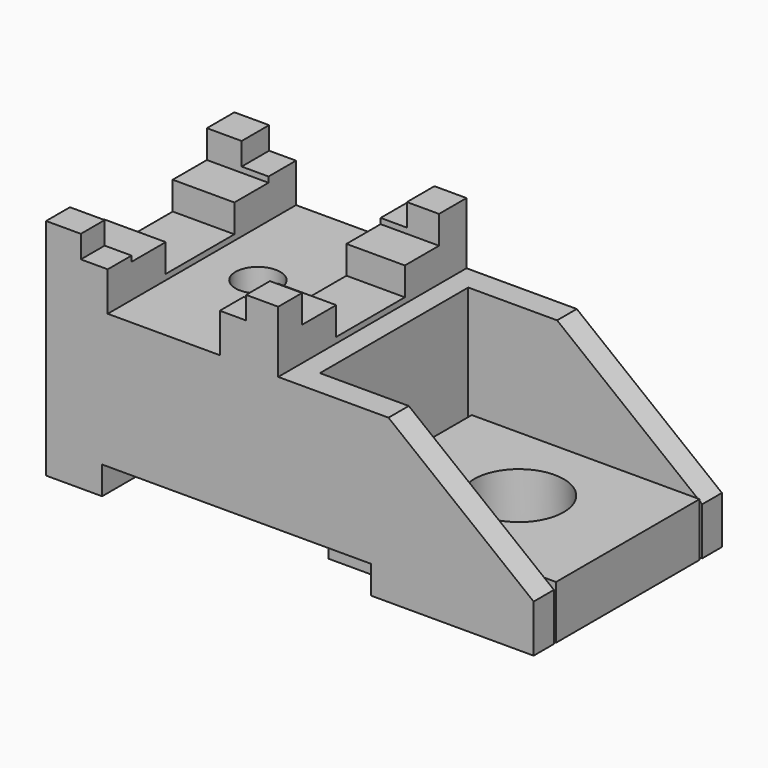
from build123d import *

# Parameters (mm, degrees)
F0_W      = 43.5
F0_H      = 20
F1_DEPTH  = 21
F2_W      = 24
F2_H      = 2.5
F2_W_2    = 2.3986939639
F2_H_2    = 2.0085112005
F2_W_3    = 2.3467258811
F3_DEPTH  = 21.001
F5_DEPTH  = 21.001
F6_R      = 2
F7_DEPTH  = 8
F9_W      = 15.2769281747
F9_H      = 2.5
F10_DEPTH = 43.501
F11_W     = 7.6569281747
F11_H     = 2.5
F12_DEPTH = 43.501
F15_DEPTH = 21.001
F16_W     = 23.7473566085
F16_H     = 16.5431026835
F17_DEPTH = 25.4
F13_W     = 20.32
F13_H     = 16
F18_DEPTH = 4.7752
F8_R      = 4
F19_DEPTH = 74
F20_R     = 4
F21_DEPTH = 4.7762


# Not quite as in the source:
# - an extrude ends at something that could not be found from the text; its depth is read off the source's solid


with BuildPart() as f1:
    # F0 (on Front) → F1 (new body)
    with BuildSketch(Plane.XZ):
        with Locations((21.75, 10)):
            Rectangle(F0_W, F0_H)
    extrude(amount=F1_DEPTH)

    # F2 (on face) → F3 (cut, through all)
    with BuildSketch(Plane.XZ.offset(21)):
        Polygon((15.5, 20), (5.5, 20), (5.5, 17.9914887995), (5.5, 14.5), (15.5, 14.5), (15.5, 17.9914887995), align=None)
        with Locations((17, 1.25)):
            Rectangle(F2_W, F2_H)
        with Locations((4.3006530181, 18.9957443997)):
            Rectangle(F2_W_2, F2_H_2)
        with Locations((16.6733629405, 18.9957443997)):
            Rectangle(F2_W_3, F2_H_2)
    extrude(amount=-F3_DEPTH, mode=Mode.SUBTRACT)

    # F4 (on face) → F5 (cut, through all)
    with BuildSketch(Plane.XZ.offset(21)):
        Polygon((43.5, 20), (23.5762298107, 20), (43.5, 4.2507629842), align=None)
    extrude(amount=-F5_DEPTH, mode=Mode.SUBTRACT)

    # F6 (on face) → F7 (cut)
    with BuildSketch(Plane.XY.offset(14.5)):
        with Locations((10.5, -10.5)):
            Circle(F6_R)
    extrude(amount=-F7_DEPTH, mode=Mode.SUBTRACT)

    # F9 (on face) → F10 (cut, through all)
    with BuildSketch(Plane(origin=(0, 0, 0), x_dir=(0, -1, 0), z_dir=(-1, 0, 0))):
        with Locations((10.7036660069, 18.75)):
            Rectangle(F9_W, F9_H)
    extrude(amount=-F10_DEPTH, mode=Mode.SUBTRACT)

    # F11 (on face) → F12 (cut, through all)
    with BuildSketch(Plane(origin=(0, 0, 0), x_dir=(0, -1, 0), z_dir=(-1, 0, 0))):
        with Locations((10.7036660069, 16.25)):
            Rectangle(F11_W, F11_H)
    extrude(amount=-F12_DEPTH, mode=Mode.SUBTRACT)

    # F14 (on face) → F15 (cut, through all)
    with BuildSketch(Plane.XZ.offset(21)):
        Polygon((23.5762298107, 20), (20.7114778459, 20), (20.7114778459, 14.4868092611), (30.5507610328, 14.4868092611), align=None)
    extrude(amount=-F15_DEPTH, mode=Mode.SUBTRACT)

    # F16 (on Top) → F17 (cut)
    with BuildSketch(Plane.XY):
        with Locations((34.4953713939, -10.4653941235)):
            Rectangle(F16_W, F16_H)
    extrude(amount=F17_DEPTH, mode=Mode.SUBTRACT)

    # F8 (on face) → F19 (cut, through all)
    with BuildSketch(Plane(origin=(0, 0, 0), x_dir=(1, 0, 0), z_dir=(0, 0, -1))):
        with Locations((36.25, 10.5)):
            Circle(F8_R)
    extrude(amount=F19_DEPTH, mode=Mode.SUBTRACT)


with BuildPart() as f18:
    # F13 (on Top) → F18 (new body)
    with BuildSketch(Plane.XY):
        with Locations((33.34, -10.5)):
            Rectangle(F13_W, F13_H)
    extrude(amount=F18_DEPTH)

    # F20 (on face) → F21 (cut, through all)
    with BuildSketch(Plane.XY.offset(4.7752)):
        with Locations((33.34, -9.9435616285)):
            Circle(F20_R)
    extrude(amount=-F21_DEPTH, mode=Mode.SUBTRACT)


solid = Compound([f1.part, f18.part])
